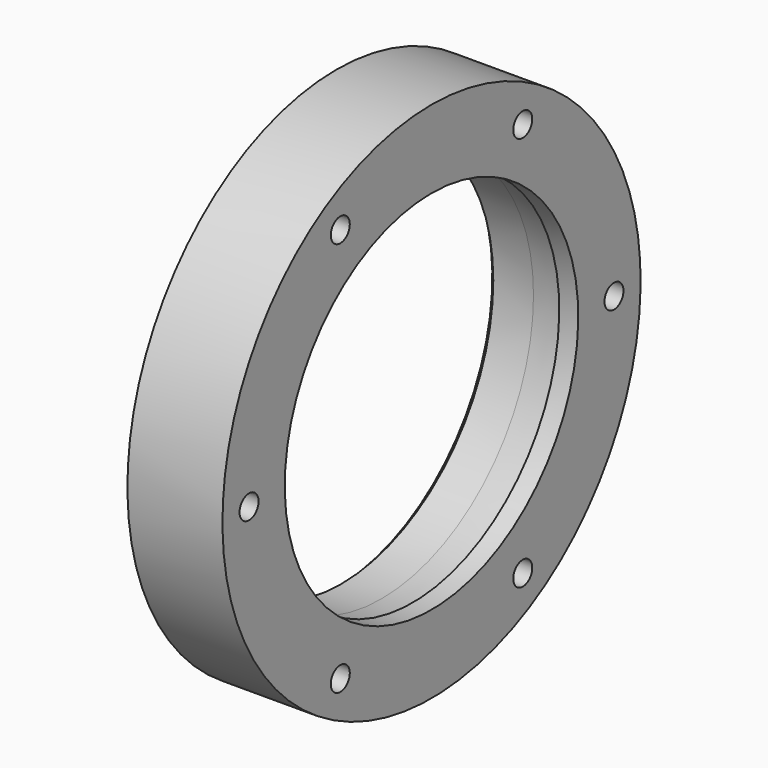
from build123d import *

# Parameters (mm, degrees)
F2_SIZE          = 1
F3_R             = 2.5
F4_DEPTH         = 20.001
F4_COPIES_COUNT  = 3
F4_COPIES_ANGLE  = 120
F4_COPIES1_COUNT = 3
F4_COPIES1_ANGLE = 120
F5_R             = 2.5
F6_DEPTH         = 20.001


# Not quite as in the source:
# - a pattern or mirror of a feature is missing from the dataset's text; its kind, count and spacing are read off the source's solid


with BuildPart() as f1:
    # F0 (on Front) → F1 (revolve)
    with BuildSketch(Plane.XZ):
        Polygon((-4, 38.6), (0, 38.6), (0, 55), (-20, 55), (-20, 40), (-10.5399421904, 40), (-4, 39.6), align=None)
    revolve(axis=Axis((12.3917190358, 0, 0), (1, 0, 0)))

    # F2
    f2_edges = [f1.edges().sort_by_distance(p)[0] for p in [
        (-20, 0, -40),
    ]]
    chamfer(f2_edges, length=F2_SIZE)

    # F3 (on face) → F4 (cut, through all)
    with BuildSketch(Plane(origin=(-20, 0, 0), x_dir=(0, -1, 0), z_dir=(-1, 0, 0))):
        with Locations((48, 0)):
            Circle(F3_R)
    f4 = extrude(amount=-F4_DEPTH, mode=Mode.SUBTRACT)

    # F4_copies: F4 ×3 about axis
    f4_copies_axis = Axis((0, 0, 0), (1, 0, 0))
    for i in range(1, F4_COPIES_COUNT):
        add(f4.rotate(f4_copies_axis, i * F4_COPIES_ANGLE / (F4_COPIES_COUNT - 1)), mode=Mode.SUBTRACT)

    # F4_copies1: F4 ×3 about axis
    f4_copies1_axis = Axis((0, 0, 0), (-1, 0, 0))
    for i in range(1, F4_COPIES1_COUNT):
        add(f4.rotate(f4_copies1_axis, i * F4_COPIES1_ANGLE / (F4_COPIES1_COUNT - 1)), mode=Mode.SUBTRACT)

    # F5 (on face) → F6 (cut, through all)
    with BuildSketch(Plane(origin=(-20, 0, 0), x_dir=(0, -1, 0), z_dir=(-1, 0, 0))):
        with Locations((-48, 0)):
            Circle(F5_R)
    extrude(amount=-F6_DEPTH, mode=Mode.SUBTRACT)


solid = f1.part
